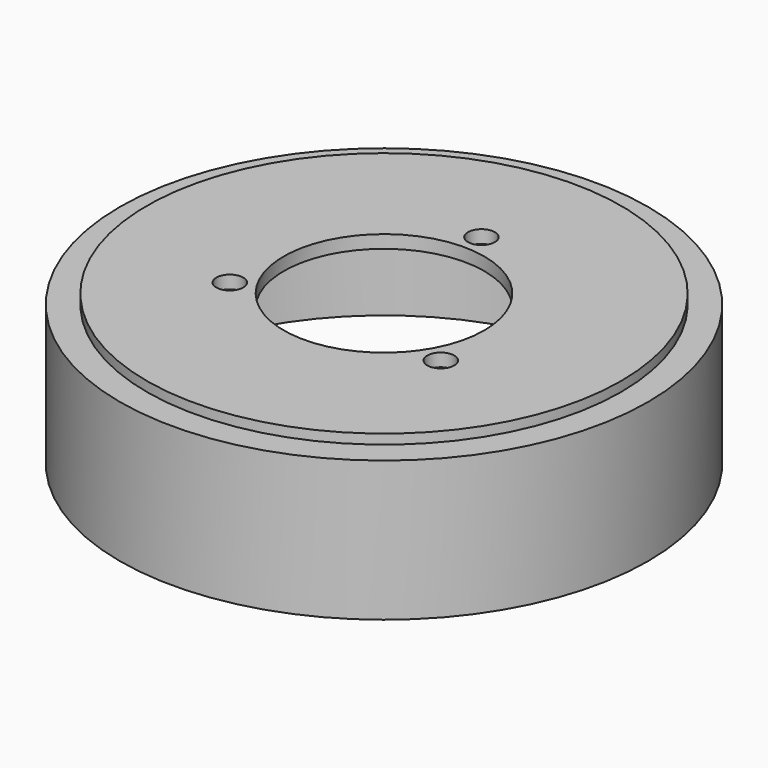
from build123d import *

# Parameters (mm, degrees)
F0_R            = 55.88
F0_R_2          = 23.622
F1_DEPTH        = 2.286
F0_R_3          = 59.055
F2_DEPTH        = 5.08
F0_R_4          = 62.23
F3_DEPTH        = 33.02
F4_R            = 3.175
F5_DEPTH        = 25.4
F5_COPIES_COUNT = 3
F7_R            = 34.1580603644
F7_R_2          = 3.175
F7_R_3          = 23.622
F8_DEPTH        = 1.524


# Not quite as in the source:
# - a pattern or mirror of a feature is missing from the dataset's text; its kind, count and spacing are read off the source's solid


with BuildPart() as f1:
    # F0 (on Top) → F1 (new body, symmetric)
    with BuildSketch(Plane.XY):
        Circle(F0_R)
        Circle(F0_R_2, mode=Mode.SUBTRACT)
    extrude(amount=F1_DEPTH, both=True)

    # F0 (on Top) → F2 (join)
    with BuildSketch(Plane.XY):
        Circle(F0_R_3)
        Circle(F0_R, mode=Mode.SUBTRACT)
    extrude(amount=-F2_DEPTH)

    # F0 (on Top) → F3 (join)
    with BuildSketch(Plane.XY):
        Circle(F0_R_4)
        Circle(F0_R_3, mode=Mode.SUBTRACT)
    extrude(amount=-F3_DEPTH)

    # F4 (on face) → F5 (cut)
    with BuildSketch(Plane.XY.offset(2.286)):
        with Locations((0, 28.702)):
            Circle(F4_R)
    f5 = extrude(amount=-F5_DEPTH, mode=Mode.SUBTRACT)

    # F5_copies: F5 ×3 about axis
    f5_copies_axis = Axis((0, 0, 0), (0, 0, 1))
    for i in range(1, F5_COPIES_COUNT):
        add(f5.rotate(f5_copies_axis, i * 360 / F5_COPIES_COUNT), mode=Mode.SUBTRACT)

    # F7 (on face) → F8 (cut)
    with BuildSketch(Plane(origin=(0, 0, -2.286), x_dir=(1, 0, 0), z_dir=(0, 0, -1))):
        Circle(F7_R)
        with Locations((0, -28.702)):
            Circle(F7_R_2, mode=Mode.SUBTRACT)
        Circle(F7_R_3, mode=Mode.SUBTRACT)
        with Locations((-24.8566611394, 14.351)):
            Circle(F7_R_2, mode=Mode.SUBTRACT)
        with Locations((24.8566611394, 14.351)):
            Circle(F7_R_2, mode=Mode.SUBTRACT)
    extrude(amount=-F8_DEPTH, mode=Mode.SUBTRACT)


solid = f1.part
